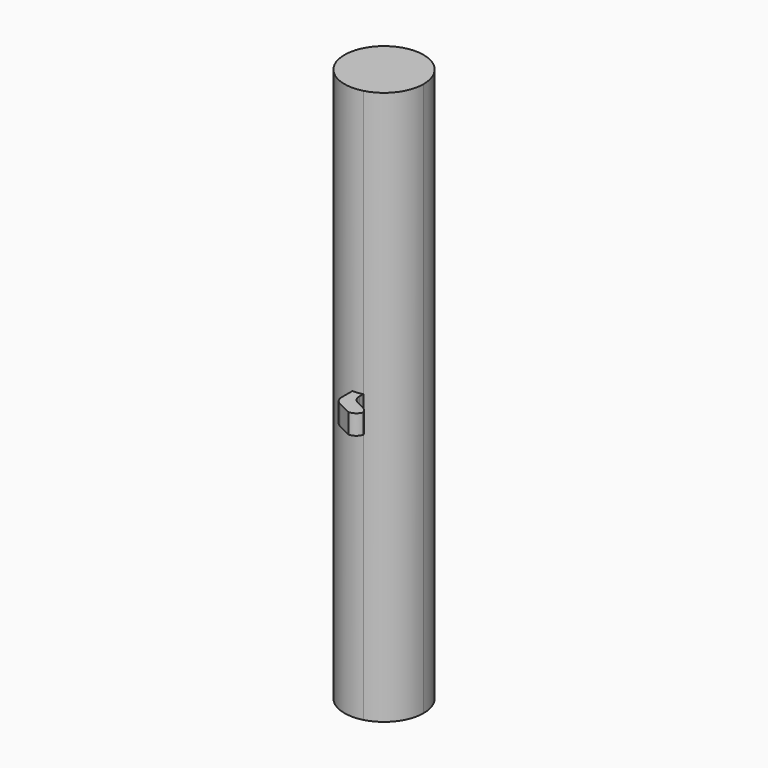
from build123d import *

# Parameters (mm, degrees)
F1_DEPTH    = 70
F2_DEPTH    = 2.5
F3_T1_DEPTH = 5
F3_T3_DEPTH = 12.6854399108
F3_T5_DEPTH = 17.5
F3_T7_DEPTH = 12.7254248594


# Not quite as in the source:
# - a fillet or chamfer that OpenCascade refuses, or shapes differently, is made with other operations: its cross-section is extruded or revolved along the edge and cut away or added


with BuildPart() as f1:
    # F0 (on Top) → F1 (new body, symmetric)
    with BuildSketch(Plane.XY):
        with BuildLine():
            ThreePointArc((2.5, -9.6824583655), (7.9056941504, -6.123724357), (10, 0))
            ThreePointArc((10, 0), (-7.0710678119, 7.0710678119), (0, -10))
            ThreePointArc((0, -10), (1.2600429248, -9.9202969627), (2.5, -9.6824583655))
        make_face()
    extrude(amount=F1_DEPTH, both=True)

    # F0 (on Top) → F2 (join, symmetric)
    with BuildSketch(Plane.XY):
        with BuildLine():
            ThreePointArc((2.5, -9.6824583655), (1.2600429248, -9.9202969627), (0, -10))
            Line((0, -10), (0, -12.4709576939))
            Line((0, -12.4709576939), (2.5, -12.4709576939))
            Line((2.5, -12.4709576939), (2.5, -9.6824583655))
        make_face()
        Polygon((2.5, -12.4709576939), (0, -12.4709576939), (0, -15), (5, -17.5), (7.5, -17.5), (7.5, -15), align=None)
    extrude(amount=F2_DEPTH, both=True)

    # F3: fillet of radius 2.5 on 4 edges, made by hand

    # F3_s2 → F3_t1 (join)
    with BuildSketch(Plane.XY.offset(-2.5)):
        with BuildLine():
            ThreePointArc((2.5, -10.9338697117), (2.8703321066, -12.2432644817), (3.871611731, -13.1647305129))
            Line((3.871611731, -13.1647305129), (2.5, -12.4709576939))
            Line((2.5, -12.4709576939), (2.5, -10.9338697117))
        make_face()
    extrude(amount=F3_T1_DEPTH)

    # F3_s4 → F3_t3 (cut)
    with BuildSketch(Plane.XY.offset(-6.3427199554)):
        with BuildLine():
            ThreePointArc((6.128388269, -14.306227181), (7.1296678934, -15.2276932122), (7.5, -16.5370879822))
            Line((7.5, -16.5370879822), (7.5, -15))
            Line((7.5, -15), (6.128388269, -14.306227181))
        make_face()
    extrude(amount=F3_T3_DEPTH, mode=Mode.SUBTRACT)

    # F3_s6 → F3_t5 (cut)
    with BuildSketch(Plane.XY.offset(-8.75)):
        with BuildLine():
            ThreePointArc((5, -17.5), (6.767766953, -16.767766953), (7.5, -15))
            Line((7.5, -15), (7.5, -17.5))
            Line((7.5, -17.5), (5, -17.5))
        make_face()
    extrude(amount=F3_T5_DEPTH, mode=Mode.SUBTRACT)

    # F3_s8 → F3_t7 (cut)
    with BuildSketch(Plane.XY.offset(-6.3627124297)):
        with BuildLine():
            ThreePointArc((0, -13.4549150281), (0.3733729791, -14.7692428084), (1.3819660113, -15.6909830056))
            Line((1.3819660113, -15.6909830056), (0, -15))
            Line((0, -15), (0, -13.4549150281))
        make_face()
    extrude(amount=F3_T7_DEPTH, mode=Mode.SUBTRACT)


solid = f1.part
